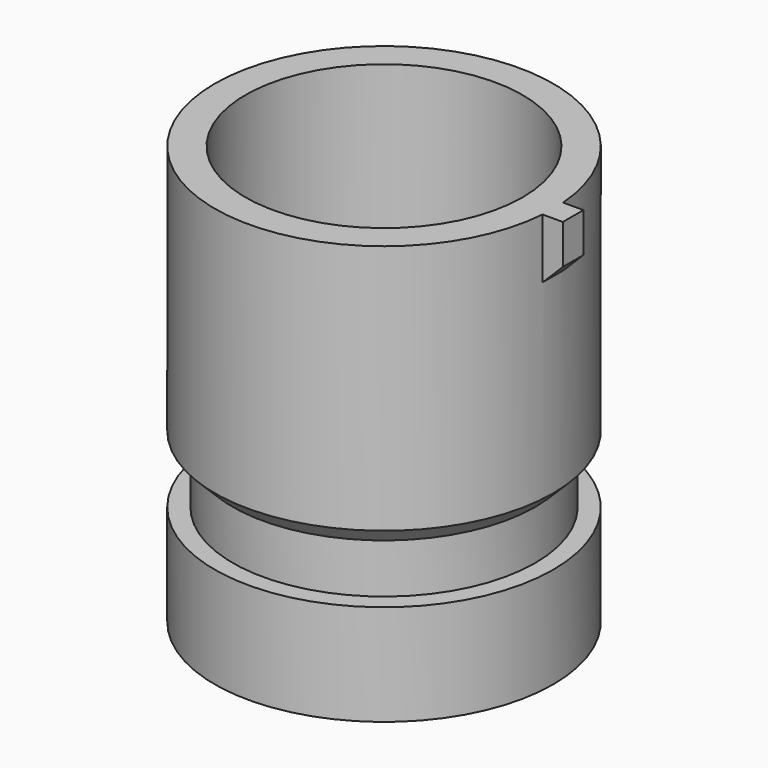
from build123d import *

# Parameters (mm, degrees)
F0_R         = 17.1
F0_R_2       = 14
F1_DEPTH     = 10.2
F2_R         = 15.275
F2_R_2       = 14
F2_R_3       = 13.275
F3_DEPTH     = 5
F4_R         = 17.1
F4_R_2       = 15.275
F4_R_3       = 14
F5_DEPTH     = 27.1
F6_S5_R      = 14
F6_T6_DEPTH  = 22
F6_S11_R     = 14
F6_T12_DEPTH = 22
F7_SIZE      = 1.8
F9_DEPTH     = 6
F10_SIZE     = 1.99999


# Not quite as in the source:
# - a fillet or chamfer that OpenCascade refuses, or shapes differently, is made with other operations: its cross-section is extruded or revolved along the edge and cut away or added
# - a fillet or chamfer is up to 0.001 mm smaller than in the source, because OpenCascade refuses the exact size


with BuildPart() as f1:
    # F0 (on Top) → F1 (new body)
    with BuildSketch(Plane.XY):
        Circle(F0_R)
        Circle(F0_R_2, mode=Mode.SUBTRACT)
    extrude(amount=F1_DEPTH)

    # F2 (on face) → F3 (join)
    with BuildSketch(Plane.XY.offset(10.2)):
        Circle(F2_R)
        Circle(F2_R_2, mode=Mode.SUBTRACT)
        Circle(F2_R_2)
        Circle(F2_R_3, mode=Mode.SUBTRACT)
    extrude(amount=F3_DEPTH)

    # F4 (on face) → F5 (join)
    with BuildSketch(Plane.XY.offset(15.2)):
        Circle(F4_R)
        Circle(F4_R_2, mode=Mode.SUBTRACT)
        Circle(F4_R_2)
        Circle(F4_R_3, mode=Mode.SUBTRACT)
    extrude(amount=F5_DEPTH)

    # F6: chamfer of 1.4 on 2 edges, made by hand


with BuildPart() as f6_tool2:
    # F6_s3 → F6_t4 (revolve)
    with BuildSketch(Plane.XZ):
        Polygon((14.675, 10.2), (13.275, 11.6), (13.275, 10.2), align=None)
    revolve(axis=Axis((0, 0, 10.2), (0, 0, 1)))

    # F6_s5 → F6_t6 (intersect, symmetric)
    with BuildSketch(Plane.XY.offset(10.9)):
        Circle(F6_S5_R)
    extrude(amount=F6_T6_DEPTH, both=True, mode=Mode.INTERSECT)


with BuildPart() as f1_1:
    add(f1.part)

    # F6_t1: cut F6_tool2
    add(f6_tool2.part, mode=Mode.SUBTRACT)


with BuildPart() as f6_tool8:
    # F6_s9 → F6_t10 (revolve)
    with BuildSketch(Plane.XZ):
        Polygon((13.275, 13.8), (14.675, 15.2), (13.275, 15.2), align=None)
    revolve(axis=Axis((0, 0, 15.2), (0, 0, 1)))

    # F6_s11 → F6_t12 (intersect, symmetric)
    with BuildSketch(Plane.XY.offset(14.5)):
        Circle(F6_S11_R)
    extrude(amount=F6_T12_DEPTH, both=True, mode=Mode.INTERSECT)


with BuildPart() as f1_2:
    add(f1_1.part)

    # F6_t7: cut F6_tool8
    add(f6_tool8.part, mode=Mode.SUBTRACT)

    # F7
    f7_edges = [f1_2.edges().sort_by_distance(p)[0] for p in [
        (-17.1, 0, 15.2),
    ]]
    chamfer(f7_edges, length=F7_SIZE)

    # F8 (on face) → F9 (join)
    with BuildSketch(Plane.XY.offset(42.3)):
        with BuildLine():
            ThreePointArc((17.0505131888, 1.3), (17.0876238185, 0.6504707804), (17.1, 0))
            Line((17.1, 0), (19.1, 0))
            Line((19.1, 0), (19.1, 1.3))
            Line((19.1, 1.3), (17.0505131888, 1.3))
        make_face()
        with BuildLine():
            Line((19.1, 0), (17.1, 0))
            ThreePointArc((17.1, 0), (17.0876238185, -0.6504707804), (17.0505131888, -1.3))
            Line((17.0505131888, -1.3), (19.1, -1.3))
            Line((19.1, -1.3), (19.1, 0))
        make_face()
        with BuildLine():
            Line((17.1, 0), (17.0505131888, 0))
            Line((17.0505131888, 0), (17.0505131888, -1.3))
            ThreePointArc((17.0505131888, -1.3), (17.0876238185, -0.6504707804), (17.1, 0))
        make_face()
        with BuildLine():
            Line((17.0505131888, 1.3), (17.0505131888, 0))
            Line((17.0505131888, 0), (17.1, 0))
            ThreePointArc((17.1, 0), (17.0876238185, 0.6504707804), (17.0505131888, 1.3))
        make_face()
    extrude(amount=-F9_DEPTH)

    # F10 (size 2 in the source; OpenCascade refuses exactly that, so slightly less here)
    f10_edges = [f1_2.edges().sort_by_distance(p)[0] for p in [
        (19.1, 0, 36.3),
    ]]
    chamfer(f10_edges, length=F10_SIZE)


solid = f1_2.part
